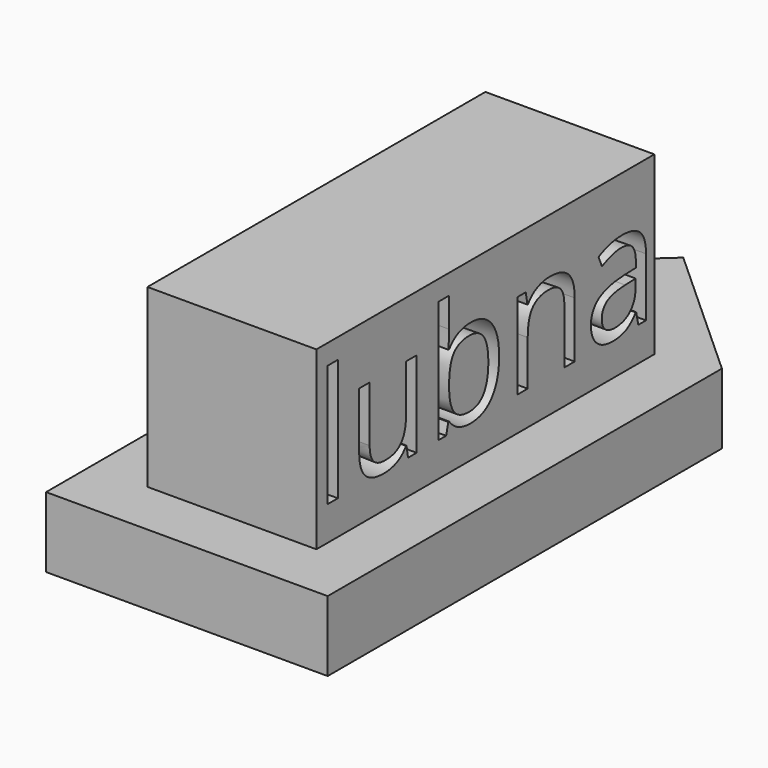
from build123d import *

# Parameters (mm, degrees)
F1_DEPTH     = 10
F2_W         = 24
F2_H         = 60
F3_DEPTH     = 25
F6_TEXT_SIZE = 22.7852607844
F7_DEPTH     = 10


# Not quite as in the source:
# - the program builds the solid bodies; features that only make, move or delete a surface that nothing else refers to are left out
# - Text() gives the source's letters only with a copy of the font that has no kerning and outlines rounded to 1/6400 em; it was checked with that copy


with BuildPart() as f1:
    # F0 (on Top) → F1 (new body)
    with BuildSketch(Plane.XY):
        Polygon((20, -24.4700775191), (20, 45.5299224809), (0, 63.6682796281), (-20, 45.5299224809), (-20, -24.4700775191), align=None)
    extrude(amount=F1_DEPTH)

    # F2 (on face) → F3 (join)
    with BuildSketch(Plane.XY.offset(10)):
        with Locations((0, 13.5299224809)):
            Rectangle(F2_W, F2_H)
    extrude(amount=F3_DEPTH)

    # F6 (on face) → F7 (cut)
    with BuildSketch(Plane.YZ.offset(12)):
        with Locations((-16.4700775191, 14.8365208963)):
            Text('lubna', F6_TEXT_SIZE, font='Open Sans', text_align=(TextAlign.LEFT, TextAlign.BOTTOM))
    extrude(amount=-F7_DEPTH, mode=Mode.SUBTRACT)


solid = f1.part
